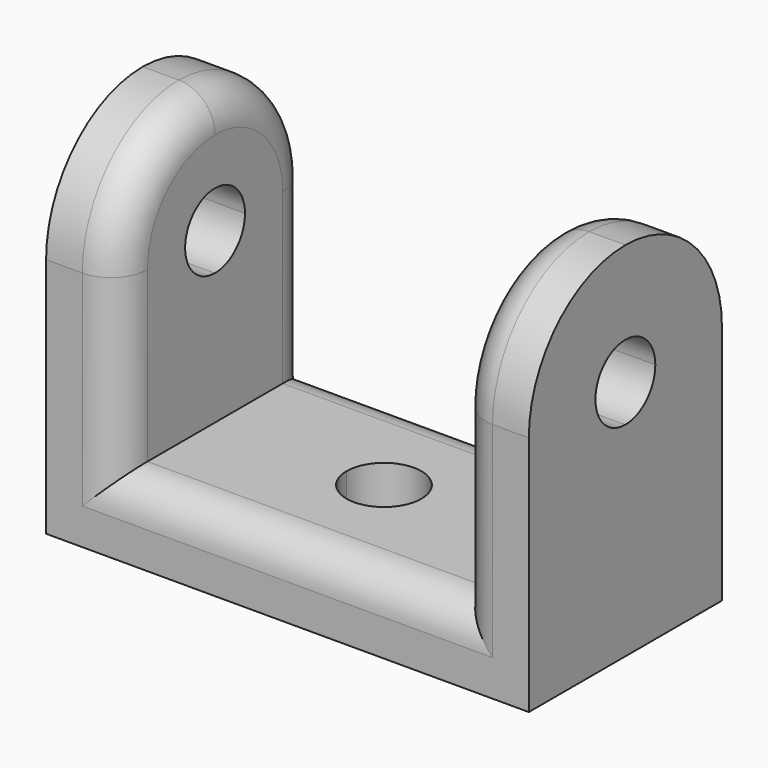
from build123d import *

# Parameters (mm, degrees)
F1_DEPTH = 3
F2_W     = 3
F2_H     = 10
F3_DEPTH = 12
F5_DEPTH = 25
F6_R     = 4.99999
F7_R     = 1.5


# Not quite as in the source:
# - a fillet or chamfer is up to 0.001 mm smaller than in the source, because OpenCascade refuses the exact size


with BuildPart() as f1:
    # F0 (on Top) → F1 (new body)
    with BuildSketch(Plane.XY):
        with BuildLine():
            Line((5.7057162493, -7.4039038014), (-2.7442837507, -7.4039038014))
            Line((-2.7442837507, -7.4039038014), (-2.7442837507, -12.4039038014))
            Line((-2.7442837507, -12.4039038014), (7.2557162493, -12.4039038014))
            Line((7.2557162493, -12.4039038014), (7.2557162493, -8.9539038014))
            ThreePointArc((7.2557162493, -8.9539038014), (6.1597007385, -8.4999193123), (5.7057162493, -7.4039038014))
        make_face()
        with BuildLine():
            Line((17.2557162493, -2.4039038014), (-2.7442837507, -2.4039038014))
            Line((-2.7442837507, -2.4039038014), (-2.7442837507, -7.4039038014))
            Line((-2.7442837507, -7.4039038014), (5.7057162493, -7.4039038014))
            ThreePointArc((5.7057162493, -7.4039038014), (7.2557162493, -5.8539038014), (8.8057162493, -7.4039038014))
            ThreePointArc((8.8057162493, -7.4039038014), (8.3517317602, -8.4999193123), (7.2557162493, -8.9539038014))
            Line((7.2557162493, -8.9539038014), (7.2557162493, -12.4039038014))
            Line((7.2557162493, -12.4039038014), (17.2557162493, -12.4039038014))
            Line((17.2557162493, -12.4039038014), (17.2557162493, -2.4039038014))
        make_face()
    extrude(amount=F1_DEPTH)

    # F2 (on face) → F3 (join)
    with BuildSketch(Plane.XY.offset(3)):
        with Locations((-1.2442837507, -7.4039038014)):
            Rectangle(F2_W, F2_H)
        with Locations((15.7557162493, -7.4039038014)):
            Rectangle(F2_W, F2_H)
    extrude(amount=F3_DEPTH)

    # F4 (on face) → F5 (cut)
    with BuildSketch(Plane(origin=(-2.7442837507, 0, 0), x_dir=(0, -1, 0), z_dir=(-1, 0, 0))):
        with BuildLine():
            ThreePointArc((5.8539038014, 10), (6.3078882906, 8.9039844892), (7.4039038014, 8.45))
            Line((7.4039038014, 8.45), (7.4039038014, 10))
            Line((7.4039038014, 10), (5.8539038014, 10))
        make_face()
        with BuildLine():
            Line((7.4039038014, 10), (7.4039038014, 8.45))
            ThreePointArc((7.4039038014, 8.45), (8.4999193123, 8.9039844892), (8.9539038014, 10))
            ThreePointArc((8.9539038014, 10), (7.4039038014, 11.55), (5.8539038014, 10))
            Line((5.8539038014, 10), (7.4039038014, 10))
        make_face()
    extrude(amount=-F5_DEPTH, mode=Mode.SUBTRACT)

    # F6 (radius 5 in the source; OpenCascade refuses exactly that, so slightly less here)
    f6_edges = [f1.edges().sort_by_distance(p)[0] for p in [
        (-1.244284, -2.403904, 15),
        (15.755716, -2.403904, 15),
        (15.755716, -12.403904, 15),
        (-1.244284, -12.403904, 15),
    ]]
    fillet(f6_edges, radius=F6_R)

    # F7
    f7_edges = [f1.edges().sort_by_distance(p)[0] for p in [
        (7.255716, -2.403904, 3),
        (7.255716, -12.403904, 3),
        (0.255716, -10.939441, 13.535537),
        (14.255716, -3.868367, 13.535537),
    ]]
    fillet(f7_edges, radius=F7_R)


solid = f1.part
